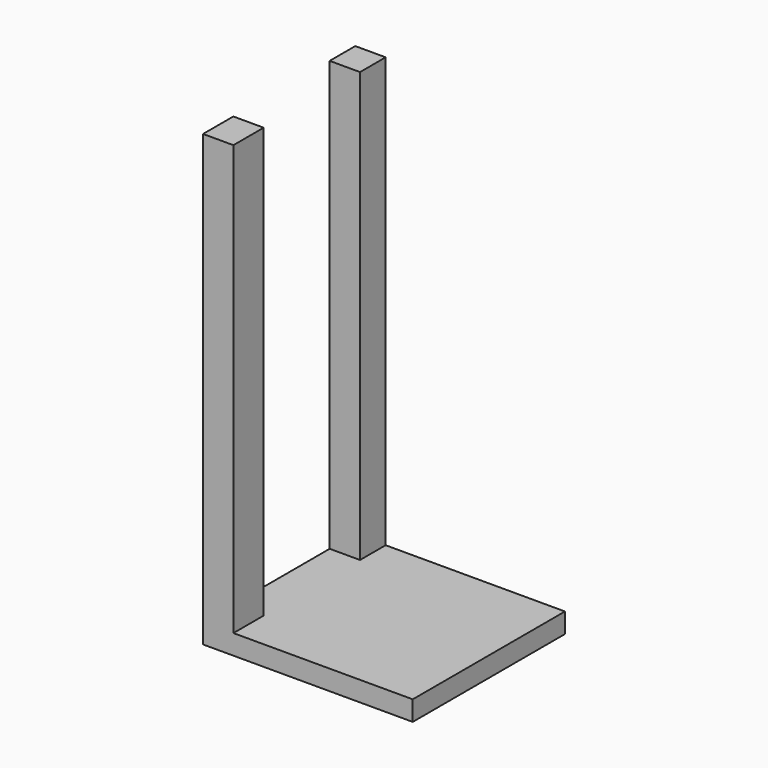
from build123d import *

# Parameters (mm, degrees)
F0_W     = 16.4634734392
F0_H     = 13.1345540285
F0_H_2   = 62.0689839125
F0_W_2   = 13.7195661664
F0_W_3   = 70.2442079782
F0_H_3   = 15.9291923046
F1_DEPTH = 9.5300190151
F2_W     = 14.5427659154
F2_H     = 15.3316706419
F2_H_2   = 18.1263536215
F3_DEPTH = 205.7239394635


# Not quite as in the source:
# - the program builds the solid bodies; features that only make, move or delete a surface that nothing else refers to are left out


with BuildPart() as f1:
    # F0 (on Top) → F1 (new body)
    with BuildSketch(Plane.XY):
        with Locations((49.1160675883, 30.5517539382)):
            Rectangle(F0_W, F0_H)
        with Locations((49.1160675883, -7.0500150323)):
            Rectangle(F0_W, F0_H_2)
        with Locations((-36.2196601927, 30.5517539382)):
            Rectangle(F0_W_2, F0_H)
        with Locations((5.7622268796, 30.5517539382)):
            Rectangle(F0_W_3, F0_H)
        with Locations((-36.2196601927, -7.0500150323)):
            Rectangle(F0_W_2, F0_H_2)
        with Locations((-36.2196601927, -46.0491031408)):
            Rectangle(F0_W_2, F0_H_3)
        with Locations((5.7622268796, -46.0491031408)):
            Rectangle(F0_W_3, F0_H_3)
        with Locations((49.1160675883, -46.0491031408)):
            Rectangle(F0_W, F0_H_3)
        with Locations((5.7622268796, -7.0500150323)):
            Rectangle(F0_W_3, F0_H_2)
    extrude(amount=F1_DEPTH)

    # F2 (on face) → F3 (join)
    with BuildSketch(Plane.XY.offset(9.5300190151)):
        with Locations((-35.8080603182, 29.4531956315)):
            Rectangle(F2_W, F2_H)
        with Locations((-35.8080603182, -44.9505224824)):
            Rectangle(F2_W, F2_H_2)
    extrude(amount=F3_DEPTH)


solid = f1.part
